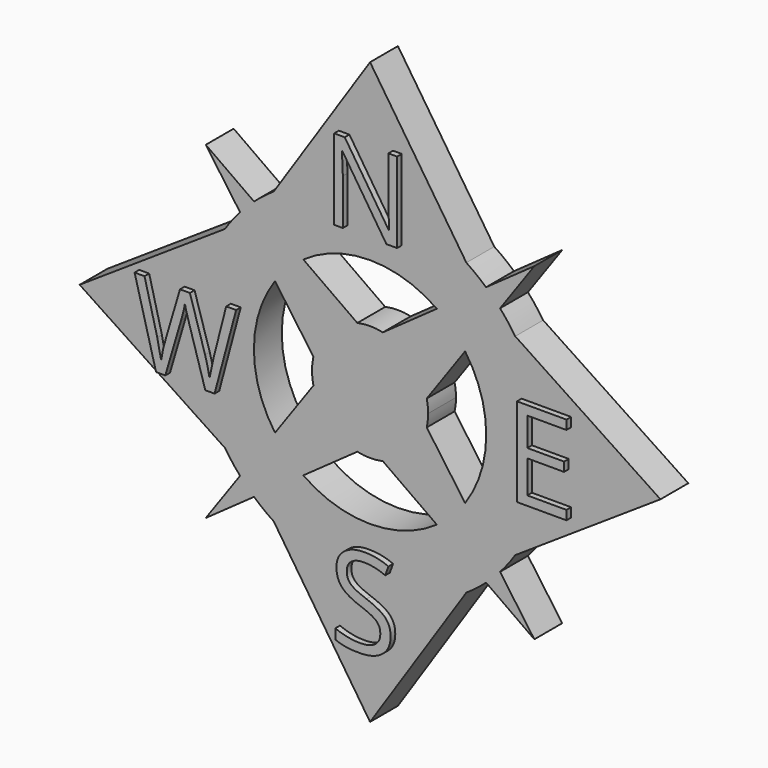
from build123d import *

# Parameters (mm, degrees)
F1_DEPTH     = 6
F2_TEXT_SIZE = 19.4275802255
F3_DEPTH     = 1
F4_TEXT_SIZE = 21.2096106048
F5_DEPTH     = 1
F6_TEXT_SIZE = 21.3927576602
F7_DEPTH     = 1
F8_TEXT_SIZE = 19.4444444444
F9_DEPTH     = 1


# Not quite as in the source:
# - Text() gives the source's letters only with a copy of the font that has no kerning and outlines rounded to 1/6400 em; it was checked with that copy


with BuildPart() as f1:
    # F0 (on Front) → F1 (new body)
    with BuildSketch(Plane.XZ):
        with BuildLine():
            ThreePointArc((-16.5831239518, 25), (0, 30), (16.5831239518, 25))
            Line((16.5831239518, 25), (0, 50))
            Line((0, 50), (-16.5831239518, 25))
        make_face()
        with BuildLine():
            ThreePointArc((-11.4985152327, 16.364111569), (0, 20), (11.4985152327, 16.364111569))
            Line((11.4985152327, 16.364111569), (19.9746579151, 22.3833206021))
            ThreePointArc((19.9746579151, 22.3833206021), (18.3256543273, 23.752271333), (16.5831239518, 25))
            ThreePointArc((16.5831239518, 25), (0, 30), (-16.5831239518, 25))
            ThreePointArc((-16.5831239518, 25), (-18.3256543273, 23.752271333), (-19.9746579151, 22.3833206021))
            Line((-19.9746579151, 22.3833206021), (-11.4985152327, 16.364111569))
        make_face()
        with BuildLine():
            ThreePointArc((-21.2132034356, 21.2132034356), (-20.6022395435, 21.8070567889), (-19.9746579151, 22.3833206021))
            Line((-19.9746579151, 22.3833206021), (-28.2842712475, 28.2842712475))
            Line((-28.2842712475, 28.2842712475), (-21.2132034356, 21.2132034356))
        make_face()
        with BuildLine():
            ThreePointArc((-22.3833206021, 19.9746579151), (-21.8070567889, 20.6022395435), (-21.2132034356, 21.2132034356))
            Line((-21.2132034356, 21.2132034356), (-28.2842712475, 28.2842712475))
            Line((-28.2842712475, 28.2842712475), (-22.3833206021, 19.9746579151))
        make_face()
        with BuildLine():
            ThreePointArc((-16.364111569, 11.4985152327), (-15.3102894042, 12.8683735709), (-14.1421356237, 14.1421356237))
            Line((-14.1421356237, 14.1421356237), (-21.2132034356, 21.2132034356))
            ThreePointArc((-21.2132034356, 21.2132034356), (-21.8070567889, 20.6022395435), (-22.3833206021, 19.9746579151))
            Line((-22.3833206021, 19.9746579151), (-16.364111569, 11.4985152327))
        make_face()
        with BuildLine():
            ThreePointArc((-14.1421356237, 14.1421356237), (-12.8683735709, 15.3102894042), (-11.4985152327, 16.364111569))
            Line((-11.4985152327, 16.364111569), (-19.9746579151, 22.3833206021))
            ThreePointArc((-19.9746579151, 22.3833206021), (-20.6022395435, 21.8070567889), (-21.2132034356, 21.2132034356))
            Line((-21.2132034356, 21.2132034356), (-14.1421356237, 14.1421356237))
        make_face()
        with BuildLine():
            ThreePointArc((-7.0710678119, 7.0710678119), (-4.8230368851, 8.7600408221), (-2.1936835012, 9.7564211008))
            Line((-2.1936835012, 9.7564211008), (-11.4985152327, 16.364111569))
            ThreePointArc((-11.4985152327, 16.364111569), (-12.8683735709, 15.3102894042), (-14.1421356237, 14.1421356237))
            Line((-14.1421356237, 14.1421356237), (-7.0710678119, 7.0710678119))
        make_face()
        with BuildLine():
            ThreePointArc((-9.7564211008, 2.1936835012), (-8.7600408221, 4.8230368851), (-7.0710678119, 7.0710678119))
            Line((-7.0710678119, 7.0710678119), (-14.1421356237, 14.1421356237))
            ThreePointArc((-14.1421356237, 14.1421356237), (-15.3102894042, 12.8683735709), (-16.364111569, 11.4985152327))
            Line((-16.364111569, 11.4985152327), (-9.7564211008, 2.1936835012))
        make_face()
        with BuildLine():
            Line((-7.0710678119, -7.0710678119), (0, 0))
            Line((0, 0), (-7.0710678119, 7.0710678119))
            ThreePointArc((-7.0710678119, 7.0710678119), (-8.7600408221, 4.8230368851), (-9.7564211008, 2.1936835012))
            ThreePointArc((-9.7564211008, 2.1936835012), (-10, 0), (-9.7564211008, -2.1936835012))
            ThreePointArc((-9.7564211008, -2.1936835012), (-8.7600408221, -4.8230368851), (-7.0710678119, -7.0710678119))
        make_face()
        with BuildLine():
            Line((0, 0), (7.0710678119, 7.0710678119))
            ThreePointArc((7.0710678119, 7.0710678119), (4.8230368851, 8.7600408221), (2.1936835012, 9.7564211008))
            ThreePointArc((2.1936835012, 9.7564211008), (0, 10), (-2.1936835012, 9.7564211008))
            ThreePointArc((-2.1936835012, 9.7564211008), (-4.8230368851, 8.7600408221), (-7.0710678119, 7.0710678119))
            Line((-7.0710678119, 7.0710678119), (0, 0))
        make_face()
        with BuildLine():
            ThreePointArc((9.7564211008, -2.1936835012), (9.9389187291, -1.1035825732), (10, 0))
            ThreePointArc((10, 0), (9.9389187291, 1.1035825732), (9.7564211008, 2.1936835012))
            ThreePointArc((9.7564211008, 2.1936835012), (8.7600408221, 4.8230368851), (7.0710678119, 7.0710678119))
            Line((7.0710678119, 7.0710678119), (0, 0))
            Line((0, 0), (7.0710678119, -7.0710678119))
            ThreePointArc((7.0710678119, -7.0710678119), (8.7600408221, -4.8230368851), (9.7564211008, -2.1936835012))
        make_face()
        with BuildLine():
            ThreePointArc((2.1936835012, -9.7564211008), (4.8230368851, -8.7600408221), (7.0710678119, -7.0710678119))
            Line((7.0710678119, -7.0710678119), (0, 0))
            Line((0, 0), (-7.0710678119, -7.0710678119))
            ThreePointArc((-7.0710678119, -7.0710678119), (-4.8230368851, -8.7600408221), (-2.1936835012, -9.7564211008))
            ThreePointArc((-2.1936835012, -9.7564211008), (0, -10), (2.1936835012, -9.7564211008))
        make_face()
        with BuildLine():
            Line((-14.1421356237, -14.1421356237), (-7.0710678119, -7.0710678119))
            ThreePointArc((-7.0710678119, -7.0710678119), (-8.7600408221, -4.8230368851), (-9.7564211008, -2.1936835012))
            Line((-9.7564211008, -2.1936835012), (-16.364111569, -11.4985152327))
            ThreePointArc((-16.364111569, -11.4985152327), (-15.3102894042, -12.8683735709), (-14.1421356237, -14.1421356237))
        make_face()
        with BuildLine():
            ThreePointArc((-2.1936835012, -9.7564211008), (-4.8230368851, -8.7600408221), (-7.0710678119, -7.0710678119))
            Line((-7.0710678119, -7.0710678119), (-14.1421356237, -14.1421356237))
            ThreePointArc((-14.1421356237, -14.1421356237), (-12.8683735709, -15.3102894042), (-11.4985152327, -16.364111569))
            Line((-11.4985152327, -16.364111569), (-2.1936835012, -9.7564211008))
        make_face()
        with BuildLine():
            ThreePointArc((-11.4985152327, -16.364111569), (-12.8683735709, -15.3102894042), (-14.1421356237, -14.1421356237))
            Line((-14.1421356237, -14.1421356237), (-21.2132034356, -21.2132034356))
            ThreePointArc((-21.2132034356, -21.2132034356), (-20.6022395435, -21.8070567889), (-19.9746579151, -22.3833206021))
            Line((-19.9746579151, -22.3833206021), (-11.4985152327, -16.364111569))
        make_face()
        with BuildLine():
            Line((-21.2132034356, -21.2132034356), (-14.1421356237, -14.1421356237))
            ThreePointArc((-14.1421356237, -14.1421356237), (-15.3102894042, -12.8683735709), (-16.364111569, -11.4985152327))
            Line((-16.364111569, -11.4985152327), (-22.3833206021, -19.9746579151))
            ThreePointArc((-22.3833206021, -19.9746579151), (-21.8070567889, -20.6022395435), (-21.2132034356, -21.2132034356))
        make_face()
        with BuildLine():
            ThreePointArc((-19.9746579151, -22.3833206021), (-20.6022395435, -21.8070567889), (-21.2132034356, -21.2132034356))
            Line((-21.2132034356, -21.2132034356), (-28.2842712475, -28.2842712475))
            Line((-28.2842712475, -28.2842712475), (-19.9746579151, -22.3833206021))
        make_face()
        with BuildLine():
            Line((-28.2842712475, -28.2842712475), (-21.2132034356, -21.2132034356))
            ThreePointArc((-21.2132034356, -21.2132034356), (-21.8070567889, -20.6022395435), (-22.3833206021, -19.9746579151))
            Line((-22.3833206021, -19.9746579151), (-28.2842712475, -28.2842712475))
        make_face()
        with BuildLine():
            Line((14.1421356237, -14.1421356237), (7.0710678119, -7.0710678119))
            ThreePointArc((7.0710678119, -7.0710678119), (4.8230368851, -8.7600408221), (2.1936835012, -9.7564211008))
            Line((2.1936835012, -9.7564211008), (11.4985152327, -16.364111569))
            ThreePointArc((11.4985152327, -16.364111569), (12.8683735709, -15.3102894042), (14.1421356237, -14.1421356237))
        make_face()
        with BuildLine():
            Line((16.364111569, -11.4985152327), (9.7564211008, -2.1936835012))
            ThreePointArc((9.7564211008, -2.1936835012), (8.7600408221, -4.8230368851), (7.0710678119, -7.0710678119))
            Line((7.0710678119, -7.0710678119), (14.1421356237, -14.1421356237))
            ThreePointArc((14.1421356237, -14.1421356237), (15.3102894042, -12.8683735709), (16.364111569, -11.4985152327))
        make_face()
        with BuildLine():
            Line((22.3833206021, -19.9746579151), (16.364111569, -11.4985152327))
            ThreePointArc((16.364111569, -11.4985152327), (15.3102894042, -12.8683735709), (14.1421356237, -14.1421356237))
            Line((14.1421356237, -14.1421356237), (21.2132034356, -21.2132034356))
            ThreePointArc((21.2132034356, -21.2132034356), (21.8070567889, -20.6022395435), (22.3833206021, -19.9746579151))
        make_face()
        with BuildLine():
            Line((21.2132034356, -21.2132034356), (14.1421356237, -14.1421356237))
            ThreePointArc((14.1421356237, -14.1421356237), (12.8683735709, -15.3102894042), (11.4985152327, -16.364111569))
            Line((11.4985152327, -16.364111569), (19.9746579151, -22.3833206021))
            ThreePointArc((19.9746579151, -22.3833206021), (20.6022395435, -21.8070567889), (21.2132034356, -21.2132034356))
        make_face()
        with BuildLine():
            Line((28.2842712475, -28.2842712475), (21.2132034356, -21.2132034356))
            ThreePointArc((21.2132034356, -21.2132034356), (20.6022395435, -21.8070567889), (19.9746579151, -22.3833206021))
            Line((19.9746579151, -22.3833206021), (28.2842712475, -28.2842712475))
        make_face()
        with BuildLine():
            Line((28.2842712475, -28.2842712475), (22.3833206021, -19.9746579151))
            ThreePointArc((22.3833206021, -19.9746579151), (21.8070567889, -20.6022395435), (21.2132034356, -21.2132034356))
            Line((21.2132034356, -21.2132034356), (28.2842712475, -28.2842712475))
        make_face()
        with BuildLine():
            ThreePointArc((19.9746579151, 22.3833206021), (20.6022395435, 21.8070567889), (21.2132034356, 21.2132034356))
            Line((21.2132034356, 21.2132034356), (28.2842712475, 28.2842712475))
            Line((28.2842712475, 28.2842712475), (19.9746579151, 22.3833206021))
        make_face()
        with BuildLine():
            ThreePointArc((21.2132034356, 21.2132034356), (21.8070567889, 20.6022395435), (22.3833206021, 19.9746579151))
            Line((22.3833206021, 19.9746579151), (28.2842712475, 28.2842712475))
            Line((28.2842712475, 28.2842712475), (21.2132034356, 21.2132034356))
        make_face()
        with BuildLine():
            ThreePointArc((11.4985152327, 16.364111569), (12.8683735709, 15.3102894042), (14.1421356237, 14.1421356237))
            Line((14.1421356237, 14.1421356237), (21.2132034356, 21.2132034356))
            ThreePointArc((21.2132034356, 21.2132034356), (20.6022395435, 21.8070567889), (19.9746579151, 22.3833206021))
            Line((19.9746579151, 22.3833206021), (11.4985152327, 16.364111569))
        make_face()
        with BuildLine():
            ThreePointArc((14.1421356237, 14.1421356237), (15.3102894042, 12.8683735709), (16.364111569, 11.4985152327))
            Line((16.364111569, 11.4985152327), (22.3833206021, 19.9746579151))
            ThreePointArc((22.3833206021, 19.9746579151), (21.8070567889, 20.6022395435), (21.2132034356, 21.2132034356))
            Line((21.2132034356, 21.2132034356), (14.1421356237, 14.1421356237))
        make_face()
        with BuildLine():
            ThreePointArc((2.1936835012, 9.7564211008), (4.8230368851, 8.7600408221), (7.0710678119, 7.0710678119))
            Line((7.0710678119, 7.0710678119), (14.1421356237, 14.1421356237))
            ThreePointArc((14.1421356237, 14.1421356237), (12.8683735709, 15.3102894042), (11.4985152327, 16.364111569))
            Line((11.4985152327, 16.364111569), (2.1936835012, 9.7564211008))
        make_face()
        with BuildLine():
            ThreePointArc((7.0710678119, 7.0710678119), (8.7600408221, 4.8230368851), (9.7564211008, 2.1936835012))
            Line((9.7564211008, 2.1936835012), (16.364111569, 11.4985152327))
            ThreePointArc((16.364111569, 11.4985152327), (15.3102894042, 12.8683735709), (14.1421356237, 14.1421356237))
            Line((14.1421356237, 14.1421356237), (7.0710678119, 7.0710678119))
        make_face()
        with BuildLine():
            Line((22.3833206021, 19.9746579151), (16.364111569, 11.4985152327))
            ThreePointArc((16.364111569, 11.4985152327), (19.0693763844, 6.0298328592), (20, 0))
            ThreePointArc((20, 0), (19.0693763844, -6.0298328592), (16.364111569, -11.4985152327))
            Line((16.364111569, -11.4985152327), (22.3833206021, -19.9746579151))
            ThreePointArc((22.3833206021, -19.9746579151), (23.752271333, -18.3256543273), (25, -16.5831239518))
            ThreePointArc((25, -16.5831239518), (28.7228132327, -8.6602540378), (30, 0))
            ThreePointArc((30, 0), (28.7228132327, 8.6602540378), (25, 16.5831239518))
            ThreePointArc((25, 16.5831239518), (23.752271333, 18.3256543273), (22.3833206021, 19.9746579151))
        make_face()
        with BuildLine():
            Line((50, 0), (25, 16.5831239518))
            ThreePointArc((25, 16.5831239518), (28.7228132327, 8.6602540378), (30, 0))
            ThreePointArc((30, 0), (28.7228132327, -8.6602540378), (25, -16.5831239518))
            Line((25, -16.5831239518), (50, 0))
        make_face()
        with BuildLine():
            Line((19.9746579151, -22.3833206021), (11.4985152327, -16.364111569))
            ThreePointArc((11.4985152327, -16.364111569), (0, -20), (-11.4985152327, -16.364111569))
            Line((-11.4985152327, -16.364111569), (-19.9746579151, -22.3833206021))
            ThreePointArc((-19.9746579151, -22.3833206021), (-18.3256543273, -23.752271333), (-16.5831239518, -25))
            ThreePointArc((-16.5831239518, -25), (0, -30), (16.5831239518, -25))
            ThreePointArc((16.5831239518, -25), (18.3256543273, -23.752271333), (19.9746579151, -22.3833206021))
        make_face()
        with BuildLine():
            Line((0, -50), (16.5831239518, -25))
            ThreePointArc((16.5831239518, -25), (0, -30), (-16.5831239518, -25))
            Line((-16.5831239518, -25), (0, -50))
        make_face()
        with BuildLine():
            Line((-22.3833206021, -19.9746579151), (-16.364111569, -11.4985152327))
            ThreePointArc((-16.364111569, -11.4985152327), (-20, 0), (-16.364111569, 11.4985152327))
            Line((-16.364111569, 11.4985152327), (-22.3833206021, 19.9746579151))
            ThreePointArc((-22.3833206021, 19.9746579151), (-23.752271333, 18.3256543273), (-25, 16.5831239518))
            ThreePointArc((-25, 16.5831239518), (-30, 0), (-25, -16.5831239518))
            ThreePointArc((-25, -16.5831239518), (-23.752271333, -18.3256543273), (-22.3833206021, -19.9746579151))
        make_face()
        with BuildLine():
            Line((-50, 0), (-25, -16.5831239518))
            ThreePointArc((-25, -16.5831239518), (-30, 0), (-25, 16.5831239518))
            Line((-25, 16.5831239518), (-50, 0))
        make_face()
    extrude(amount=F1_DEPTH)

    # F2 (on face) → F3 (join)
    with BuildSketch(Plane.XZ.offset(6)):
        with Locations((-7.2842712475, 24)):
            Text('N', F2_TEXT_SIZE, font='Open Sans', text_align=(TextAlign.LEFT, TextAlign.BOTTOM))
    extrude(amount=F3_DEPTH)

    # F4 (on face) → F5 (join)
    with BuildSketch(Plane.XZ.offset(6)):
        with Locations((-6.2842712475, -39.2709196355)):
            Text('S', F4_TEXT_SIZE, font='Open Sans', text_align=(TextAlign.LEFT, TextAlign.BOTTOM))
    extrude(amount=F5_DEPTH)

    # F6 (on face) → F7 (join)
    with BuildSketch(Plane.XZ.offset(6)):
        with Locations((24, -7.7842712475)):
            Text('E', F6_TEXT_SIZE, font='Open Sans', text_align=(TextAlign.LEFT, TextAlign.BOTTOM))
    extrude(amount=F7_DEPTH)

    # F8 (on face) → F9 (join)
    with BuildSketch(Plane.XZ.offset(6)):
        with Locations((-39.9978298611, -8.2842712475)):
            Text('W', F8_TEXT_SIZE, font='Open Sans', text_align=(TextAlign.LEFT, TextAlign.BOTTOM))
    extrude(amount=F9_DEPTH)


solid = f1.part
